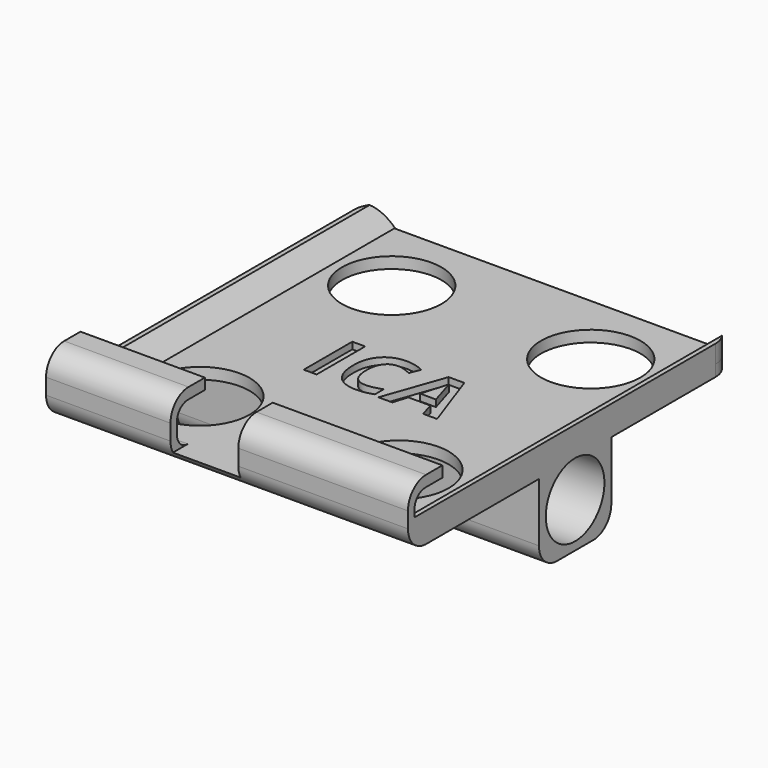
from build123d import *

# Parameters (mm, degrees)
F0_W          = 80
F0_H          = 90
F1_DEPTH      = 2.5
F2_W          = 80
F2_H          = 9.5
F3_DEPTH      = 11
F4_W          = 7.7
F4_H          = 8.5892867669
F5_DEPTH      = 90
F6_R          = 5
F7_W          = 80
F7_H          = 20
F8_DEPTH      = 18
F9_R          = 8.1
F10_DEPTH     = 90
F11_R         = 5
F12_R         = 3
F13_R         = 1.25
F14_DEPTH     = 5
F15_R         = 11
F16_DEPTH     = 25
F17_TEXT_SIZE = 18.796994118
F18_DEPTH     = 1.5
F19_W         = 5
F19_H         = 89.1964286566
F19_H_2       = 89.3156333847
F20_DEPTH     = 4
F21_R         = 4.9999
F22_SIZE      = 3.99999
F23_W         = 15
F23_H         = 18.636355854
F24_DEPTH     = 25


# Not quite as in the source:
# - a fillet or chamfer is up to 0.001 mm smaller than in the source, because OpenCascade refuses the exact size
# - Text() gives the source's letters only with a copy of the font that has no kerning and outlines rounded to 1/6400 em; it was checked with that copy


with BuildPart() as f1:
    # F0 (on Top) → F1 (new body)
    with BuildSketch(Plane.XY):
        with Locations((7.3676436394, -9.8051031729)):
            Rectangle(F0_W, F0_H)
    extrude(amount=F1_DEPTH)

    # F2 (on face) → F3 (join)
    with BuildSketch(Plane.XY.offset(2.5)):
        with Locations((7.3676436394, -50.0551031729)):
            Rectangle(F2_W, F2_H)
    extrude(amount=F3_DEPTH)

    # F4 (on face) → F5 (cut)
    with BuildSketch(Plane(origin=(-32.6323563606, 0, 0), x_dir=(0, -1, 0), z_dir=(-1, 0, 0))):
        with Locations((49.1551031729, 6.7946433835)):
            Rectangle(F4_W, F4_H)
    extrude(amount=-F5_DEPTH, mode=Mode.SUBTRACT)

    # F6
    f6_edges = [f1.edges().sort_by_distance(p)[0] for p in [
        (7.367644, -54.805103, 13.5),
        (7.367644, -54.805103, 0),
    ]]
    fillet(f6_edges, radius=F6_R)

    # F7 (on face) → F8 (join)
    with BuildSketch(Plane(origin=(0, 0, 0), x_dir=(1, 0, 0), z_dir=(0, 0, -1))):
        with Locations((7.3676436394, 8.6191175412)):
            Rectangle(F7_W, F7_H)
    extrude(amount=F8_DEPTH)

    # F9 (on face) → F10 (cut)
    with BuildSketch(Plane(origin=(-32.6323563606, 0, 0), x_dir=(0, -1, 0), z_dir=(-1, 0, 0))):
        with Locations((8.6191175412, -8.1)):
            Circle(F9_R)
    extrude(amount=-F10_DEPTH, mode=Mode.SUBTRACT)

    # F11
    f11_edges = [f1.edges().sort_by_distance(p)[0] for p in [
        (7.367644, -18.619118, -18),
        (7.367644, 1.380882, -18),
        (47.367644, 35.194897, 1.25),
        (-32.632356, 35.194897, 1.25),
    ]]
    fillet(f11_edges, radius=F11_R)

    # F12
    f12_edges = [f1.edges().sort_by_distance(p)[0] for p in [
        (7.367644, -53.005103, 11.089287),
        (7.367644, -53.005103, 2.5),
    ]]
    fillet(f12_edges, radius=F12_R)

    # F13 (on face) → F14 (cut)
    with BuildSketch(Plane(origin=(0, 0, -18), x_dir=(1, 0, 0), z_dir=(0, 0, -1))):
        with Locations((-11.6323563606, 8.6191175412)):
            Circle(F13_R)
        with Locations((26.3676436394, 8.6191175412)):
            Circle(F13_R)
    extrude(amount=-F14_DEPTH, mode=Mode.SUBTRACT)

    # F15 (on face) → F16 (cut)
    with BuildSketch(Plane.XY.offset(2.5)):
        with Locations((-14.6323563606, 18.1948968271)):
            Circle(F15_R)
        with Locations((29.3676436394, 18.1948968271)):
            Circle(F15_R)
        with Locations((-14.6323563606, -34.8051031729)):
            Circle(F15_R)
        with Locations((29.3676436394, -34.8051031729)):
            Circle(F15_R)
    extrude(amount=-F16_DEPTH, mode=Mode.SUBTRACT)

    # F17 (on face) → F18 (cut)
    with BuildSketch(Plane.XY.offset(2.5)):
        with Locations((-8.5386002902, -15.8422177192)):
            Text('ICA', F17_TEXT_SIZE, font='Open Sans', font_style=FontStyle.BOLD, text_align=(TextAlign.LEFT, TextAlign.BOTTOM))
    extrude(amount=-F18_DEPTH, mode=Mode.SUBTRACT)

    # F19 (on face) → F20 (join)
    with BuildSketch(Plane.XY.offset(2.5)):
        with Locations((-30.1323563606, -9.2410705984)):
            Rectangle(F19_W, F19_H)
        with Locations((44.8676436394, -9.4629198652)):
            Rectangle(F19_W, F19_H_2)
    extrude(amount=F20_DEPTH)

    # F21 (radius 5 in the source; OpenCascade refuses exactly that, so slightly less here)
    f21_edges = [f1.edges().sort_by_distance(p)[0] for p in [
        (-32.632356, 35.357144, 4.5),
        (47.367644, 35.194897, 4.5),
    ]]
    fillet(f21_edges, radius=F21_R)

    # F22 (call 1 of 2: OpenCascade refuses the feature's edges together) (size 4 in the source; OpenCascade refuses exactly that, so slightly less here)
    f22_edges = [f1.edges().sort_by_distance(p)[0] for p in [
        (-27.632356, -8.82398, 6.5),
    ]]
    chamfer(f22_edges, length=F22_SIZE)

    # F22#2 (call 2 of 2) (size 4 in the source; OpenCascade refuses exactly that, so slightly less here)
    f22_2_edges = [f1.edges().sort_by_distance(p)[0] for p in [
        (42.367644, -8.905103, 6.5),
    ]]
    chamfer(f22_2_edges, length=F22_SIZE)

    # F23 (on face) → F24 (cut)
    with BuildSketch(Plane.XY.offset(2.5)):
        with Locations((2.3676436394, -50.1428600401)):
            Rectangle(F23_W, F23_H)
    extrude(amount=F24_DEPTH, mode=Mode.SUBTRACT)


solid = f1.part
